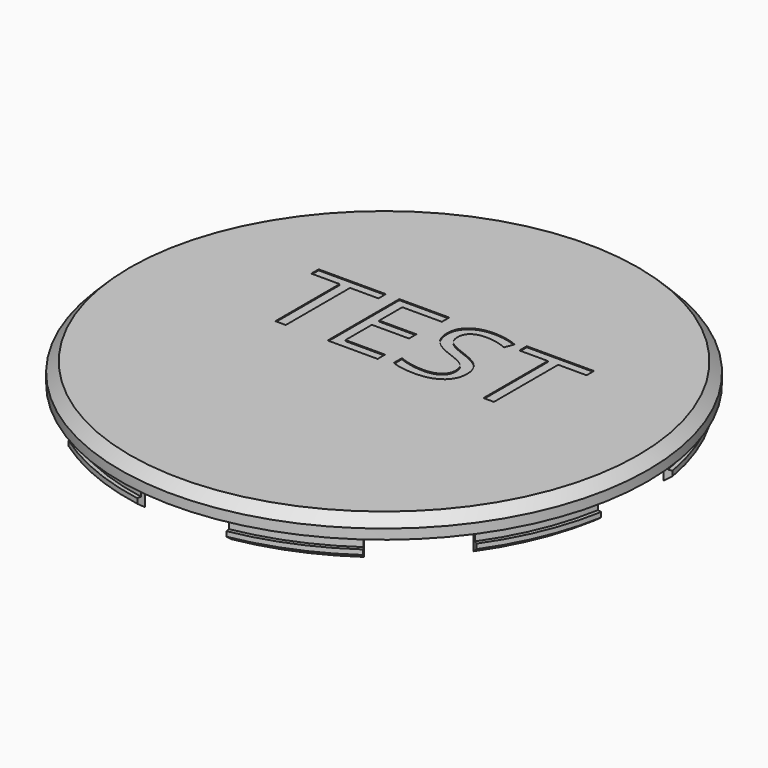
from build123d import *

# Parameters (mm, degrees)
F0_R         = 34
F1_DEPTH     = 2.54
F2_SIZE      = 1.27
F6_DEPTH     = 25.4
F7_TEXT_SIZE = 16.1680483466
F8_DEPTH     = 0.127


# Not quite as in the source:
# - Text() gives the source's letters only with a copy of the font that has no kerning and outlines rounded to 1/6400 em; it was checked with that copy


with BuildPart() as f1:
    # F0 (on Top) → F1 (new body)
    with BuildSketch(Plane.XY):
        Circle(F0_R)
    extrude(amount=F1_DEPTH)

    # F2
    f2_edges = [f1.edges().sort_by_distance(p)[0] for p in [
        (-34, 0, 2.54),
    ]]
    chamfer(f2_edges, length=F2_SIZE)

    # F3 (on Front) → F4 (revolve)
    with BuildSketch(Plane.XZ):
        Polygon((32.558478415, -1.6122375382), (32.558478415, 0), (32.0019163191, 0), (32.0019163191, -3.015749855), (33.0666489899, -2.2413982078), (33.0666489899, -1.6122375382), align=None)
    revolve(axis=Axis((0, 0, -9.7409160808), (0, 0, -1)))

    # F5 (on Top) → F6 (cut)
    with BuildSketch(Plane.XY):
        with BuildLine():
            Line((-6.0419374232, 34.2655298634), (0, 0))
            Line((0, 0), (6.0419374232, 34.2655298634))
            ThreePointArc((6.0419374232, 34.2655298634), (0, 34.7941308937), (-6.0419374232, 34.2655298634))
        make_face()
        with BuildLine():
            Line((-28.5016834508, 19.9570936039), (0, 0))
            Line((0, 0), (-19.9570936039, 28.5016834508))
            ThreePointArc((-19.9570936039, 28.5016834508), (-24.6031659004, 24.6031659004), (-28.5016834508, 19.9570936039))
        make_face()
        with BuildLine():
            Line((-34.2655298634, -6.0419374232), (0, 0))
            Line((0, 0), (-34.2655298634, 6.0419374232))
            ThreePointArc((-34.2655298634, 6.0419374232), (-34.7941308937, 0), (-34.2655298634, -6.0419374232))
        make_face()
        with BuildLine():
            Line((-19.9570936039, -28.5016834508), (0, 0))
            Line((0, 0), (-28.5016834508, -19.9570936039))
            ThreePointArc((-28.5016834508, -19.9570936039), (-24.6031659004, -24.6031659004), (-19.9570936039, -28.5016834508))
        make_face()
        with BuildLine():
            Line((6.0419374232, -34.2655298634), (0, 0))
            Line((0, 0), (-6.0419374232, -34.2655298634))
            ThreePointArc((-6.0419374232, -34.2655298634), (0, -34.7941308937), (6.0419374232, -34.2655298634))
        make_face()
        with BuildLine():
            Line((28.5016834508, -19.9570936039), (0, 0))
            Line((0, 0), (19.9570936039, -28.5016834508))
            ThreePointArc((19.9570936039, -28.5016834508), (24.6031659004, -24.6031659004), (28.5016834508, -19.9570936039))
        make_face()
        with BuildLine():
            Line((34.2655298634, 6.0419374232), (0, 0))
            Line((0, 0), (34.2655298634, -6.0419374232))
            ThreePointArc((34.2655298634, -6.0419374232), (34.7941308937, 0), (34.2655298634, 6.0419374232))
        make_face()
        with BuildLine():
            Line((19.9570936039, 28.5016834508), (0, 0))
            Line((0, 0), (28.5016834508, 19.9570936039))
            ThreePointArc((28.5016834508, 19.9570936039), (24.6031659004, 24.6031659004), (19.9570936039, 28.5016834508))
        make_face()
    extrude(amount=-F6_DEPTH, mode=Mode.SUBTRACT)

    # F7 (on face) → F8 (cut)
    with BuildSketch(Plane.XY.offset(2.54)):
        with Locations((-17.8025369842, 0)):
            Text('TEST', F7_TEXT_SIZE, font='Open Sans', text_align=(TextAlign.LEFT, TextAlign.BOTTOM))
    extrude(amount=-F8_DEPTH, mode=Mode.SUBTRACT)


solid = f1.part
